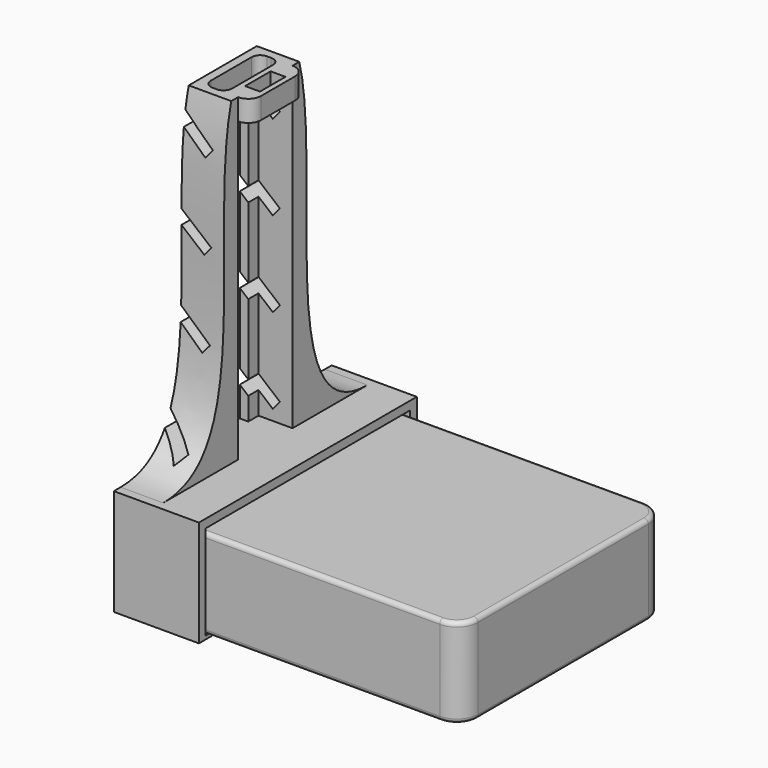
from build123d import *

# Parameters (mm, degrees)
F0_W      = 80
F0_H      = 60
F0_R      = 2.5
F1_DEPTH  = 21
F2_R      = 5
F3_R      = 1
F5_DEPTH  = 10
F6_DEPTH  = 1.7
F7_W      = 20
F7_H      = 0.8
F7_H_2    = 22.2
F8_DEPTH  = 2
F9_DEPTH  = 60
F10_W     = 20
F10_H     = 2
F10_H_2   = 22.2
F10_H_3   = 0.8
F11_DEPTH = 2
F13_DEPTH = 25
F14_W     = 8
F14_H     = 16
F15_DEPTH = 75
F16_W     = 16
F16_H     = 5
F17_DEPTH = 3
F18_R     = 2.99999
F19_W     = 3.5
F19_H     = 7.5
F20_DEPTH = 5
F21_W     = 10
F21_H     = 67
F22_DEPTH = 25
F23_DEPTH = 2
F24_DEPTH = 2
F25_R     = 2


# Not quite as in the source:
# - a fillet or chamfer is up to 0.001 mm smaller than in the source, because OpenCascade refuses the exact size


with BuildPart() as f1:
    # F0 (on Top) → F1 (new body)
    with BuildSketch(Plane.XY):
        with Locations((40, 30)):
            Rectangle(F0_W, F0_H)
        with Locations((10, 10)):
            Circle(F0_R, mode=Mode.SUBTRACT)
        with Locations((70, 10)):
            Circle(F0_R, mode=Mode.SUBTRACT)
        with Locations((10, 50)):
            Circle(F0_R, mode=Mode.SUBTRACT)
        with Locations((70, 50)):
            Circle(F0_R, mode=Mode.SUBTRACT)
        with Locations((10, 10)):
            Circle(F0_R)
        with Locations((70, 10)):
            Circle(F0_R)
        with Locations((70, 50)):
            Circle(F0_R)
        with Locations((10, 50)):
            Circle(F0_R)
    extrude(amount=F1_DEPTH)

    # F2
    f2_edges = [f1.edges().sort_by_distance(p)[0] for p in [
        (0, 0, 10.5),
        (80, 0, 10.5),
        (80, 60, 10.5),
        (0, 60, 10.5),
    ]]
    fillet(f2_edges, radius=F2_R)

    # F3
    f3_edges = [f1.edges().sort_by_distance(p)[0] for p in [
        (40, 0, 21),
        (40, 0, 0),
        (0, 30, 0),
        (0, 30, 21),
        (1.464466, 58.535534, 0),
        (1.464466, 1.464466, 0),
        (78.535534, 58.535534, 0),
        (78.535534, 1.464466, 0),
        (80, 30, 0),
        (1.464466, 58.535534, 21),
        (1.464466, 1.464466, 21),
        (78.535534, 58.535534, 21),
        (78.535534, 1.464466, 21),
        (80, 30, 21),
    ]]
    fillet(f3_edges, radius=F3_R)

    # F4 (on face) → F5 (cut)
    with BuildSketch(Plane(origin=(0, 60, 0), x_dir=(-1, 0, 0), z_dir=(0, 1, 0))):
        with BuildLine():
            Line((-35.25, 13.25), (-44.75, 13.25))
            ThreePointArc((-44.75, 13.25), (-45.4571067812, 12.9571067812), (-45.75, 12.25))
            Line((-45.75, 12.25), (-45.75, 8.75))
            ThreePointArc((-45.75, 8.75), (-45.4571067812, 8.0428932188), (-44.75, 7.75))
            Line((-44.75, 7.75), (-35.25, 7.75))
            ThreePointArc((-35.25, 7.75), (-34.5428932188, 8.0428932188), (-34.25, 8.75))
            Line((-34.25, 8.75), (-34.25, 12.25))
            ThreePointArc((-34.25, 12.25), (-34.5428932188, 12.9571067812), (-35.25, 13.25))
        make_face()
    extrude(amount=-F5_DEPTH, mode=Mode.SUBTRACT)

    # F0 (on Top) → F6 (join)
    with BuildSketch(Plane.XY):
        with Locations((10, 10)):
            Circle(F0_R)
        with Locations((70, 10)):
            Circle(F0_R)
        with Locations((70, 50)):
            Circle(F0_R)
        with Locations((10, 50)):
            Circle(F0_R)
    extrude(amount=-F6_DEPTH)


with BuildPart() as f8:
    # F7 (on Front) → F8 (new body)
    with BuildSketch(Plane.XZ):
        with Locations((10, -0.6)):
            Rectangle(F7_W, F7_H)
        Polygon((0, 24), (0, 22), (20, 22), (20, 24), (10, 24), align=None)
        with Locations((10, 10.9)):
            Rectangle(F7_W, F7_H_2)
    extrude(amount=F8_DEPTH)

    # F7 (on Front) → F9 (join, through all)
    with BuildSketch(Plane.XZ):
        Polygon((0, 24), (0, 22), (20, 22), (20, 24), (10, 24), align=None)
        Polygon((0, 31), (0, 24), (10, 24), (10, 99), (0, 99), (0, 94.3940589523), (7.033558887, 88.4922022843), (5.3623111018, 86.5004867322), (0, 91), (0, 74.3940589523), (7.033558887, 68.4922022843), (5.3623111018, 66.5004867322), (0, 71), (0, 54.3940589523), (7.033558887, 48.4922022843), (5.3623111018, 46.5004867322), (0, 51), (0, 34.3940589523), (7.033558887, 28.4922022843), (5.3623111018, 26.5004867322), align=None)
    extrude(amount=-F9_DEPTH)

    # F10 (on face) → F11 (join)
    with BuildSketch(Plane(origin=(0, 60, 0), x_dir=(-1, 0, 0), z_dir=(0, 1, 0))):
        with Locations((-10, 23)):
            Rectangle(F10_W, F10_H)
        with Locations((-10, 10.9)):
            Rectangle(F10_W, F10_H_2)
        with Locations((-10, -0.6)):
            Rectangle(F10_W, F10_H_3)
    extrude(amount=F11_DEPTH)

    # F12 (on face) → F13 (cut)
    with BuildSketch(Plane.YZ.offset(10)):
        with BuildLine():
            Line((0, 99), (0, 24))
            add(Edge.make_bspline(
                [(20, 99), (13.3333333333, 74), (27.1956510843, 24), (0, 24)],
                knots=[0, 0, 0, 0, 77.6208734813, 77.6208734813, 77.6208734813, 77.6208734813], degree=3))
            Line((20, 99), (3e-10, 99))
        make_face()
        with BuildLine():
            add(Edge.make_bspline(
                [(40, 99), (46.6666666667, 74), (32.8043489157, 24), (60, 24)],
                knots=[0, 0, 0, 0, 77.6208734813, 77.6208734813, 77.6208734813, 77.6208734813], degree=3))
            Line((60, 24), (60, 99))
            Line((60, 99), (40, 99))
        make_face()
    extrude(amount=-F13_DEPTH, mode=Mode.SUBTRACT)

    # F14 (on face) → F15 (cut, through all)
    with BuildSketch(Plane.XY.offset(99)):
        with Locations((6, 30)):
            Rectangle(F14_W, F14_H)
    extrude(amount=-F15_DEPTH, mode=Mode.SUBTRACT)

    # F16 (on face) → F17 (join, symmetric)
    with BuildSketch(Plane.YZ.offset(10)):
        with Locations((30, 96.5)):
            Rectangle(F16_W, F16_H)
    extrude(amount=F17_DEPTH, both=True)

    # F18 (radius 3 in the source; OpenCascade refuses exactly that, so slightly less here)
    f18_edges = [f8.edges().sort_by_distance(p)[0] for p in [
        (13, 22, 96.5),
        (13, 38, 96.5),
    ]]
    fillet(f18_edges, radius=F18_R)

    # F19 (on face) → F20 (cut, through all)
    with BuildSketch(Plane.XY.offset(99)):
        with Locations((10, 30)):
            Rectangle(F19_W, F19_H)
    extrude(amount=-F20_DEPTH, mode=Mode.SUBTRACT)

    # F21 (on face) → F22 (cut)
    with BuildSketch(Plane(origin=(0, 0, 0), x_dir=(0, -1, 0), z_dir=(-1, 0, 0))):
        with Locations((-30, 57.5)):
            Rectangle(F21_W, F21_H)
    extrude(amount=-F22_DEPTH, mode=Mode.SUBTRACT)

    # F7 (on Front) → F23 (join)
    with BuildSketch(Plane.XZ):
        with Locations((10, -0.6)):
            Rectangle(F7_W, F7_H)
    extrude(amount=-F23_DEPTH)

    # F10 (on face) → F24 (join)
    with BuildSketch(Plane(origin=(0, 60, 0), x_dir=(-1, 0, 0), z_dir=(0, 1, 0))):
        with Locations((-10, -0.6)):
            Rectangle(F10_W, F10_H_3)
    extrude(amount=-F24_DEPTH)

    # F25
    f25_edges = [f8.edges().sort_by_distance(p)[0] for p in [
        (7, 38, 96.5),
        (2, 38, 95.85793),
        (2, 22, 95.85793),
        (7, 22, 96.5),
    ]]
    fillet(f25_edges, radius=F25_R)


solid = Compound([f1.part, f8.part])
